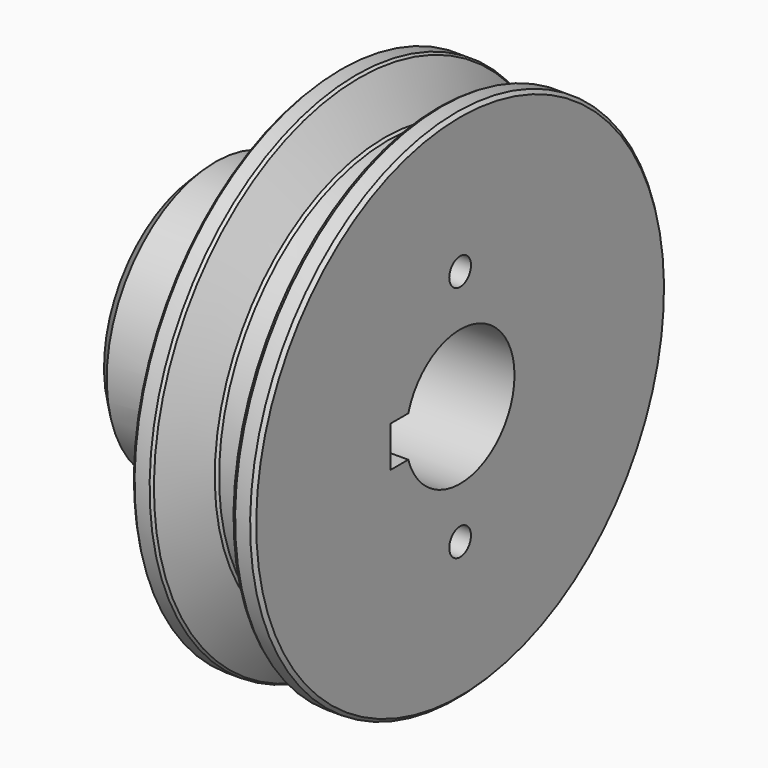
from build123d import *

# Parameters (mm, degrees)
F3_SIZE   = 1
F6_DEPTH  = 19
F8_D      = 2.5
F8_DEPTH  = 14.2
F8_TIP    = 0.7510757738
F10_D     = 2
F10_DEPTH = 6
F10_TIP   = 0.600860619


# Not quite as in the source:
# - a fillet or chamfer that OpenCascade refuses, or shapes differently, is made with other operations: its cross-section is extruded or revolved along the edge and cut away or added


with BuildPart() as f2:
    # F0 (on Front) → F2 (revolve)
    with BuildSketch(Plane.XZ):
        Polygon((0, 10), (0, 0), (19, 0), (19, 19), (17.5, 19), (15.4792740578, 15.5), (13.5207259422, 15.5), (11.5, 19), (10, 19), (10, 10), align=None)
    revolve(axis=Axis((9.5, 0, 0), (-1, 0, 0)))

    # F3
    f3_edges = [f2.edges().sort_by_distance(p)[0] for p in [
        (0, 0, -10),
    ]]
    chamfer(f3_edges, length=F3_SIZE)

    # F4: chamfer of 0.25 on 10 edges, made by hand

    # F4_s1 → F4_t2 (revolve)
    with BuildSketch(Plane.XZ):
        Polygon((9.75, 10), (10, 10.25), (10, 10), align=None)
    revolve(axis=Axis((10, 0, 0), (-1, 0, 0)))

    # F4_s3 → F4_t4 (revolve)
    with BuildSketch(Plane.XZ):
        Polygon((15.3349364905, 15.5), (15.5514428415, 15.625), (15.4792740578, 15.5), align=None)
    revolve(axis=Axis((15.4792740578, 0, 0), (-1, 0, 0)))

    # F4_s5 → F4_t6 (revolve)
    with BuildSketch(Plane.XZ):
        Polygon((13.4485571585, 15.625), (13.6650635095, 15.5), (13.5207259422, 15.5), align=None)
    revolve(axis=Axis((13.5207259422, 0, 0), (-1, 0, 0)))

    # F4_s7 → F4_t8 (revolve, cut)
    with BuildSketch(Plane.XZ):
        Polygon((11.3556624327, 19), (11.5721687836, 18.875), (11.5, 19), align=None)
    revolve(axis=Axis((11.5, 0, 0), (-1, 0, 0)), mode=Mode.SUBTRACT)

    # F4_s9 → F4_t10 (revolve, cut)
    with BuildSketch(Plane.XZ):
        Polygon((10, 18.75), (10.25, 19), (10, 19), align=None)
    revolve(axis=Axis((10, 0, 0), (-1, 0, 0)), mode=Mode.SUBTRACT)

    # F4_s11 → F4_t12 (revolve, cut)
    with BuildSketch(Plane.XZ):
        Polygon((18.75, 19), (19, 18.75), (19, 19), align=None)
    revolve(axis=Axis((19, 0, 0), (-1, 0, 0)), mode=Mode.SUBTRACT)

    # F4_s13 → F4_t14 (revolve, cut)
    with BuildSketch(Plane.XZ):
        Polygon((17.4278312164, 18.875), (17.6443375673, 19), (17.5, 19), align=None)
    revolve(axis=Axis((17.5, 0, 0), (-1, 0, 0)), mode=Mode.SUBTRACT)

    # F5 (on Right) → F6 (cut, through all)
    with BuildSketch(Plane.YZ):
        with BuildLine():
            Line((-6.4, -1.5), (-4.7696960071, -1.5))
            ThreePointArc((-4.7696960071, -1.5), (5, 0), (-4.7696960071, 1.5))
            Line((-4.7696960071, 1.5), (-6.4, 1.5))
            Line((-6.4, 1.5), (-6.4, -1.5))
        make_face()
    extrude(amount=F6_DEPTH, mode=Mode.SUBTRACT)

    # F8
    with Locations(Plane.XZ.offset(10)):
        with Locations((5, 0)):
            Hole(F8_D / 2, depth=F8_DEPTH)
            with Locations((0, 0, -(F8_DEPTH + F8_TIP / 2))):  # 118° drill point
                Cone(0, F8_D / 2, F8_TIP, mode=Mode.SUBTRACT)

    # F10
    with Locations(Plane.YZ.offset(19)):
        with Locations((0, 8.75), (0, -8.75)):
            Hole(F10_D / 2, depth=F10_DEPTH)
            with Locations((0, 0, -(F10_DEPTH + F10_TIP / 2))):  # 118° drill point
                Cone(0, F10_D / 2, F10_TIP, mode=Mode.SUBTRACT)


solid = f2.part
